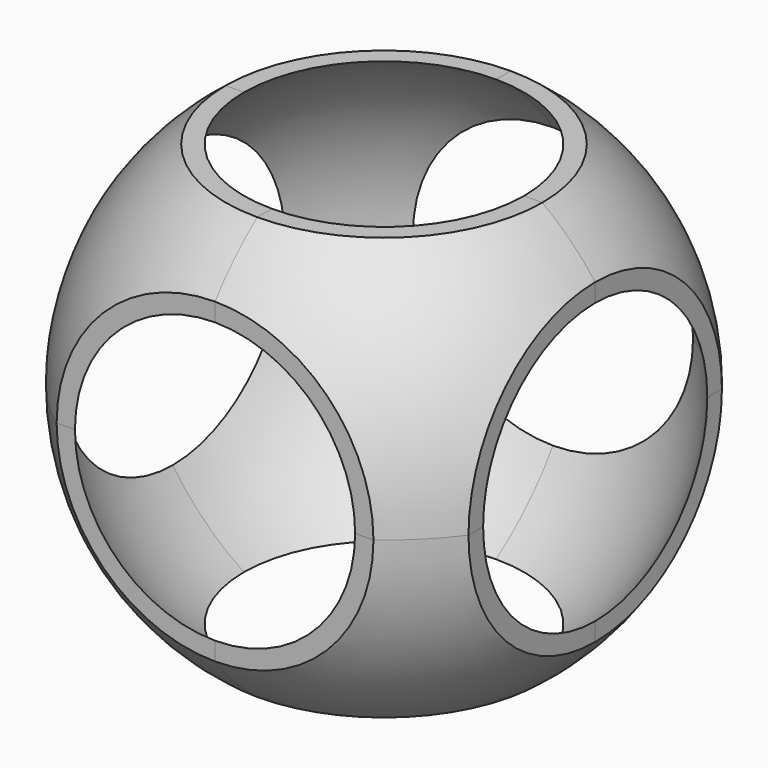
from build123d import *

# Parameters (mm, degrees)
F1_ANGLE      = 90
F2_W          = 9.8706889153
F2_H          = 16.293104738
F2_W_2        = 21.0186052322
F2_H_2        = 47.4185418094
F2_W_3        = 22.7245930582
F2_H_3        = 6.0117966682
F2_W_4        = 26.1547192931
F2_H_4        = 39.7323071957
F3_DEPTH      = 79
F3_DEPTH_BACK = 25.001
F4_W          = 20
F4_H          = 20
F5_DEPTH      = 20.001
F7_COUNT      = 4


# Not quite as in the source:
# - an extrude ends at something that could not be found from the text; its depth is read off the source's solid


with BuildPart() as f1:
    # F0 (on Front) → F1 (revolve)
    with BuildSketch(Plane.XZ):
        with BuildLine():
            Line((0, -24), (0, -25))
            ThreePointArc((0, -25), (25, 0), (0, 25))
            Line((0, 25), (0, 24))
            ThreePointArc((0, 24), (24, 0), (0, -24))
        make_face()
    revolve(axis=Axis((0, 0, 24.5), (0, 0, -1)), revolution_arc=F1_ANGLE)

    # F2 (on Front) → F3 (cut, two sides)
    with BuildSketch(Plane.XZ) as f3_sk:
        Polygon((62.8828846811, -47.4185418094), (62.8828846811, 46.2751645351), (20, 46.2751645351), (20, 36.293104738), (29.8706889153, 36.293104738), (29.8706889153, 20), (20, 20), (20, 0), (41.0186052322, 0), (41.0186052322, -47.4185418094), align=None)
        with Locations((24.9353444576, 28.146552369)):
            Rectangle(F2_W, F2_H)
        Polygon((20, 20), (20, 36.293104738), (-22.7245930582, 36.293104738), (-22.7245930582, 26.0117966682), (0, 26.0117966682), (0, 20), align=None)
        Polygon((41.0186052322, -54.5961894095), (41.0186052322, -47.4185418094), (20, -47.4185418094), (20, 0), (0, 0), (0, -39.7323071957), (-26.1547192931, -39.7323071957), (-26.1547192931, -54.5961894095), align=None)
        with Locations((30.5093026161, -23.7092709047)):
            Rectangle(F2_W_2, F2_H_2)
        Polygon((0, 0), (0, 20), (-22.7245930582, 20), (-22.7245930582, 26.0117966682), (-45.8779521286, 26.0117966682), (-45.8779521286, -39.7323071957), (-26.1547192931, -39.7323071957), (-26.1547192931, 0), align=None)
        with Locations((-11.3622965291, 23.0058983341)):
            Rectangle(F2_W_3, F2_H_3)
        with Locations((-13.0773596466, -19.8661535978)):
            Rectangle(F2_W_4, F2_H_4)
    extrude(amount=-F3_DEPTH, mode=Mode.SUBTRACT)
    extrude(f3_sk.sketch, amount=F3_DEPTH_BACK, mode=Mode.SUBTRACT)

    # F4 (on Right) → F5 (intersect, through all)
    with BuildSketch(Plane.YZ):
        with Locations((-10, 10)):
            Rectangle(F4_W, F4_H)
    extrude(amount=F5_DEPTH, mode=Mode.INTERSECT)


with BuildPart() as f6_1:
    # F6: instance of F1
    add(f1.part.mirror(Plane.XY))


with BuildPart() as f7_1:
    # F7: instance of F1
    add(f1.part.rotate(Axis((0, 0, 24.5), (0, 0, -1)), 1 * 360 / F7_COUNT))


with BuildPart() as f7_2:
    # F7: instance of F1
    add(f1.part.rotate(Axis((0, 0, 24.5), (0, 0, -1)), 2 * 360 / F7_COUNT))


with BuildPart() as f7_3:
    # F7: instance of F1
    add(f1.part.rotate(Axis((0, 0, 24.5), (0, 0, -1)), 3 * 360 / F7_COUNT))


with BuildPart() as f7_4:
    # F7: instance of F6_1
    add(f6_1.part.rotate(Axis((0, 0, 24.5), (0, 0, -1)), 1 * 360 / F7_COUNT))


with BuildPart() as f7_5:
    # F7: instance of F6_1
    add(f6_1.part.rotate(Axis((0, 0, 24.5), (0, 0, -1)), 2 * 360 / F7_COUNT))


with BuildPart() as f7_6:
    # F7: instance of F6_1
    add(f6_1.part.rotate(Axis((0, 0, 24.5), (0, 0, -1)), 3 * 360 / F7_COUNT))


solid = Compound([f1.part, f6_1.part, f7_1.part, f7_2.part, f7_3.part, f7_4.part, f7_5.part, f7_6.part])
